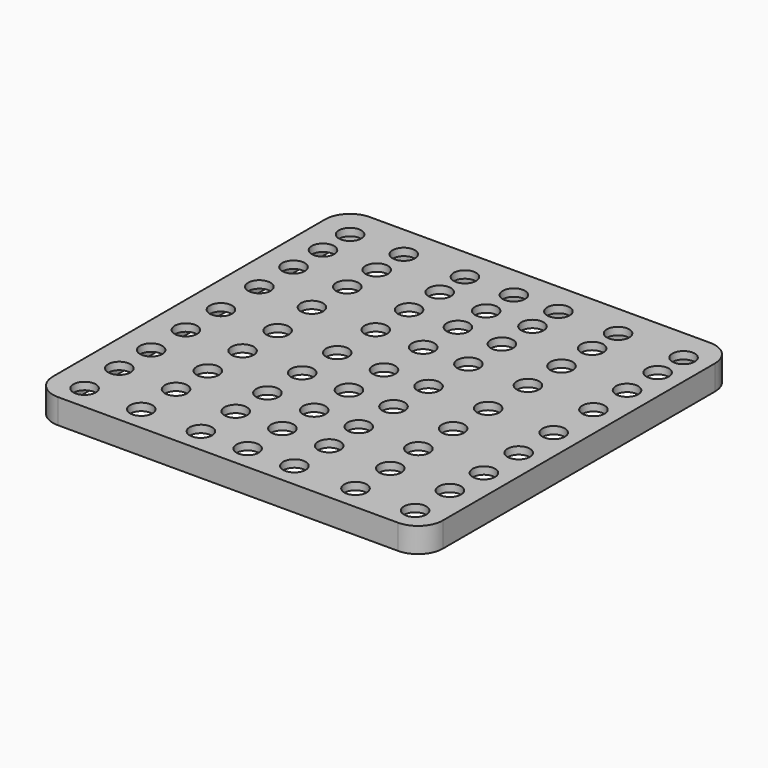
from build123d import *

# Parameters (mm, degrees)
F0_W           = 157
F0_H           = 157
F1_DEPTH       = 10
F2_W           = 151
F2_H           = 151
F3_DEPTH       = 7
F5_D           = 9
F5_CSINK_D     = 10
F5_CSINK_ANGLE = 90
F6_R           = 10
F7_R           = 10
F8_R           = 10


# Not quite as in the source:
# - a feature names something its author has since deleted; it is built from what else it names


with BuildPart() as f1:
    # F0 (on Top) → F1 (new body)
    with BuildSketch(Plane.XY):
        Rectangle(F0_W, F0_H)
    extrude(amount=F1_DEPTH)

    # F2 (on Top) → F3 (cut)
    with BuildSketch(Plane.XY):
        Rectangle(F2_W, F2_H)
    extrude(amount=F3_DEPTH, mode=Mode.SUBTRACT)

    # F5 (through all)
    with Locations(Plane(origin=(0, 0, 0), x_dir=(1, 0, 0), z_dir=(0, 0, -1))):
        with Locations((0, 0), (0, -19.7167731822), (0, -37.2098498046), (0, -51.4415055513), (0, -65.3766617179), (17.9378120229, 0), (41.9537350535, 0), (68.3415979147, 0), (-18.8272930682, 0), (-42.8432114422, 0), (-65.6731575727, 0), (0, 17.6413226873), (0, 35.1343974471), (0, 51.1450096965), (41.9537350535, -36.9133576751), (68.3415979147, -65.3766617179), (68.3415979147, -52.3309856653), (68.3415979147, -36.9133576751), (68.3415979147, -20.0132653117), (18.234308809, -19.7167731822), (17.9378120229, -36.9133576751), (41.9537350535, -52.3309856653), (41.9537350535, -65.3766617179), (17.9378120229, -52.3309856653), (-19.7167731822, -65.3766617179), (-65.9696534276, -65.3766617179), (17.9378120229, -65.3766617179), (41.9537350535, -20.0132653117), (-19.4202791899, -52.3309856653), (-19.4202791899, -36.9133576751), (-19.1237870604, -19.7167731822), (-65.9696534276, -19.7167731822), (-65.9696534276, -36.9133576751), (-65.9696534276, -51.7380014062), (-44.3256758153, -51.7380014062), (-44.3256758153, -36.9133576751), (-44.3256758153, -19.123788923), (-44.3256758153, -65.3766617179), (-65.6731575727, 68.638086319), (-65.6731575727, 51.1450096965), (-65.6731575727, 35.1343974471), (-65.6731575727, 17.6413226873), (-42.8432114422, 17.6413226873), (-42.8432114422, 35.1343974471), (-18.8272930682, 35.1343974471), (-18.8272930682, 17.6413226873), (-42.8432114422, 68.638086319), (-18.8272930682, 68.638086319), (-18.8272930682, 51.1450096965), (18.8272949308, 51.1450096965), (17.9378120229, 35.1343974471), (17.9378120229, 17.6413226873), (41.9537350535, 17.6413226873), (68.3415979147, 17.6413226873), (68.3415979147, 35.1343974471), (41.9537350535, 35.1343974471), (43.4361994267, 51.1450096965), (18.8272949308, 68.638086319), (0, 68.638086319), (43.4361994267, 68.638086319), (67.4521178007, 68.638086319), (67.4521178007, 51.1450096965), (-42.8432114422, 51.1450096965)):
            CounterSinkHole(F5_D / 2, F5_CSINK_D / 2, counter_sink_angle=F5_CSINK_ANGLE)

    # F6
    f6_edges = [f1.edges().sort_by_distance(p)[0] for p in [
        (78.5, 78.5, 5),
        (-78.5, 78.5, 5),
        (78.5, -78.5, 5),
    ]]
    fillet(f6_edges, radius=F6_R)

    # F7
    f7_edges = [f1.edges().sort_by_distance(p)[0] for p in [
        (-78.5, -78.5, 5),
    ]]
    fillet(f7_edges, radius=F7_R)

    # F8
    f8_edges = [f1.edges().sort_by_distance(p)[0] for p in [
        (75.5, -75.5, 3.5),
        (-75.5, -75.5, 3.5),
        (-75.5, 75.5, 3.5),
        (75.5, 75.5, 3.5),
    ]]
    fillet(f8_edges, radius=F8_R)


solid = f1.part
